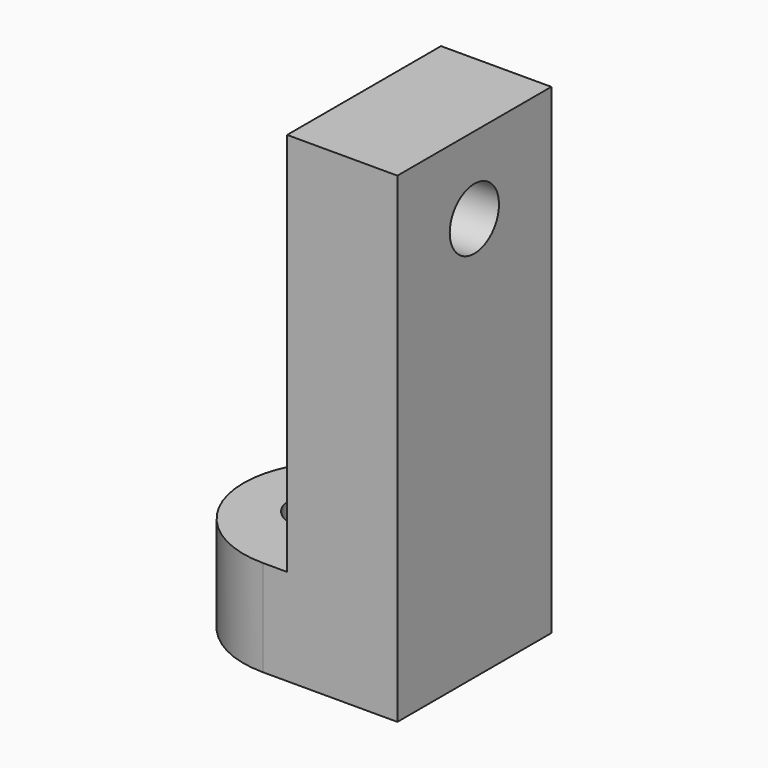
from build123d import *

# Parameters (mm, degrees)
F0_W     = 12
F0_H     = 10
F1_DEPTH = 5
F2_W     = 5.7338950146
F2_H     = 10
F3_DEPTH = 20
F4_R     = 1.6
F5_DEPTH = 10
F6_R     = 1.6
F7_DEPTH = 10
F8_R     = 4.99999


# Not quite as in the source:
# - a fillet or chamfer is up to 0.001 mm smaller than in the source, because OpenCascade refuses the exact size


with BuildPart() as f1:
    # F0 (on Top) → F1 (new body)
    with BuildSketch(Plane.XY):
        Rectangle(F0_W, F0_H)
    extrude(amount=F1_DEPTH)

    # F2 (on face) → F3 (join)
    with BuildSketch(Plane.XY.offset(5)):
        with Locations((3.1330524927, 0)):
            Rectangle(F2_W, F2_H)
    extrude(amount=F3_DEPTH)

    # F4 (on face) → F5 (cut)
    with BuildSketch(Plane(origin=(0.2661049854, 0, 0), x_dir=(0, -1, 0), z_dir=(-1, 0, 0))):
        with Locations((0, 21)):
            Circle(F4_R)
    extrude(amount=-F5_DEPTH, mode=Mode.SUBTRACT)

    # F6 (on face) → F7 (cut)
    with BuildSketch(Plane.XY.offset(5)):
        with Locations((-2, 0)):
            Circle(F6_R)
    extrude(amount=-F7_DEPTH, mode=Mode.SUBTRACT)

    # F8 (radius 5 in the source; OpenCascade refuses exactly that, so slightly less here)
    f8_edges = [f1.edges().sort_by_distance(p)[0] for p in [
        (-6, -5, 2.5),
        (-6, 5, 2.5),
    ]]
    fillet(f8_edges, radius=F8_R)


solid = f1.part
